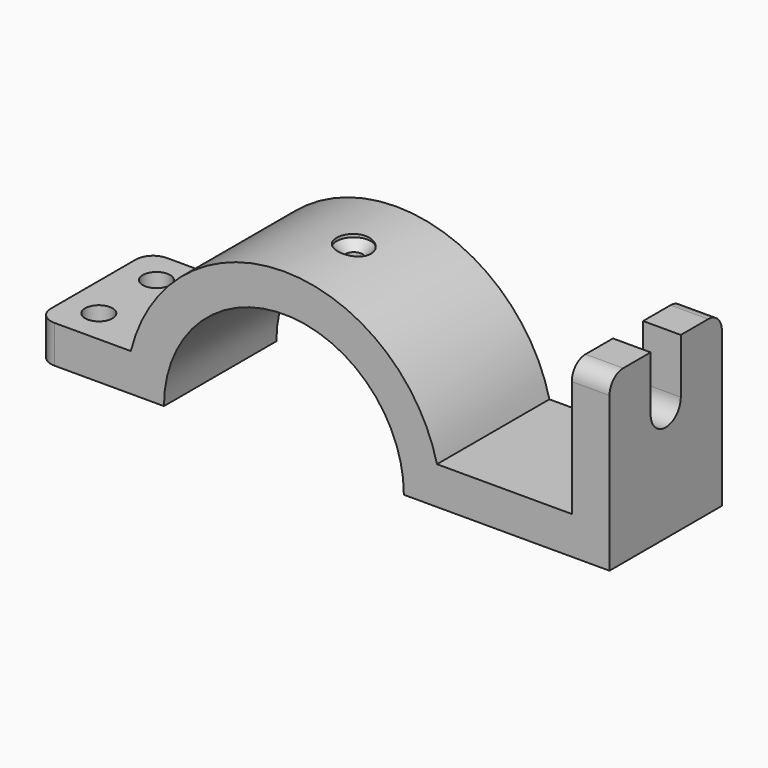
from build123d import *

# Parameters (mm, degrees)
F0_W           = 26
F0_H           = 11
F0_W_2         = 38
F1_DEPTH       = 20.5
F2_R           = 5
F3_R           = 5
F4_R           = 4
F5_DEPTH       = 12
F7_DEPTH       = 25
F9_D           = 5
F9_START       = 4.8890258
F9_CSINK_D     = 10
F9_CSINK_ANGLE = 90


# Not quite as in the source:
# - a feature names something its author has since deleted; it is built from what else it names


with BuildPart() as f1:
    # F0 (on Front) → F1 (new body, symmetric)
    with BuildSketch(Plane.XZ):
        with Locations((-84.2427663654, 5.5)):
            Rectangle(F0_W, F0_H)
        with BuildLine():
            Line((-69.9081892337, 11), (-71.2427663654, 11))
            Line((-71.2427663654, 11), (-71.2427663654, 0))
            ThreePointArc((-71.2427663654, 0), (-70.9079032421, 5.5403315812), (-69.9081892337, 11))
        make_face()
        with BuildLine():
            ThreePointArc((-69.9081892337, 11), (-70.9079032421, 5.5403315812), (-71.2427663654, 0))
            Line((-71.2427663654, 0), (-60.2427663654, 0))
            ThreePointArc((-60.2427663654, 0), (-25.2427663654, 35), (9.7572336346, 0))
            Line((9.7572336346, 0), (20.7572336346, 0))
            ThreePointArc((20.7572336346, 0), (20.4223705113, 5.5403315812), (19.4226565028, 11))
            ThreePointArc((19.4226565028, 11), (-25.2427663654, 46), (-69.9081892337, 11))
        make_face()
        with BuildLine():
            ThreePointArc((19.4226565028, 11), (20.4223705113, 5.5403315812), (20.7572336346, 0))
            Line((20.7572336346, 0), (20.7572336346, 11))
            Line((20.7572336346, 11), (19.4226565028, 11))
        make_face()
        with Locations((39.7572336346, 5.5)):
            Rectangle(F0_W_2, F0_H)
        Polygon((58.7572336346, 11), (58.7572336346, 0), (69.7572336346, 0), (69.7572336346, 50), (58.7572336346, 50), align=None)
    extrude(amount=F1_DEPTH, both=True)

    # F2
    f2_edges = [f1.edges().sort_by_distance(p)[0] for p in [
        (-97.242766, -20.5, 5.5),
        (-97.242766, 20.5, 5.5),
    ]]
    fillet(f2_edges, radius=F2_R)

    # F3
    f3_edges = [f1.edges().sort_by_distance(p)[0] for p in [
        (64.257234, -20.5, 50),
        (64.257234, 20.5, 50),
    ]]
    fillet(f3_edges, radius=F3_R)

    # F4 (on face) → F5 (cut)
    with BuildSketch(Plane.XY.offset(11)):
        with Locations((-87.2427663654, 10.5)):
            Circle(F4_R)
        with Locations((-87.2427663654, -10.5)):
            Circle(F4_R)
    extrude(amount=-F5_DEPTH, mode=Mode.SUBTRACT)

    # F6 (on face) → F7 (cut)
    with BuildSketch(Plane.YZ.offset(69.7572336346)):
        with BuildLine():
            Line((5.5, 50), (-5.5, 50))
            Line((-5.5, 50), (-5.5, 45))
            Line((-5.5, 45), (-5.5, 34))
            ThreePointArc((-5.5, 34), (0, 39.5), (5.5, 34))
            Line((5.5, 34), (5.5, 45))
            Line((5.5, 45), (5.5, 50))
        make_face()
        with BuildLine():
            ThreePointArc((5.5, 34), (0, 39.5), (-5.5, 34))
            Line((-5.5, 34), (5.5, 34))
        make_face()
        with BuildLine():
            Line((5.5, 34), (-5.5, 34))
            ThreePointArc((-5.5, 34), (0, 28.5), (5.5, 34))
        make_face()
    extrude(amount=-F7_DEPTH, mode=Mode.SUBTRACT)

    # F9 (through all)
    # its depths count from where the whole tool has entered the part; down to there all is cleared
    with Locations(Plane.XY.offset(50).offset(-F9_START)):
        with Locations((-21.2427663654, 0)):
            CounterSinkHole(F9_D / 2, F9_CSINK_D / 2, counter_sink_angle=F9_CSINK_ANGLE)


solid = f1.part
